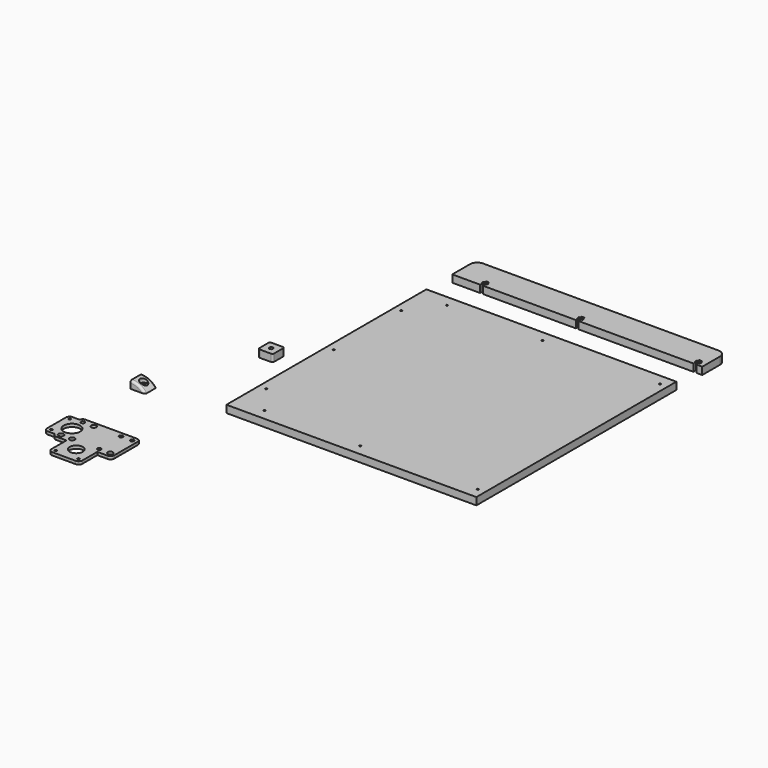
from build123d import *

# Parameters (mm, degrees)
F0_R          = 3.555
F0_R_2        = 1.5
F0_R_3        = 9
F0_R_4        = 11.2
F0_R_5        = 2.5
F1_DEPTH      = 4
F0_W          = 340
F0_H          = 340
F2_DEPTH      = 10
F6_DEPTH      = 39.1
F6_DEPTH_BACK = 25
F0_W_2        = 20
F0_H_2        = 20
F0_R_6        = 5
F8_DEPTH      = 10
F9_DEPTH      = 4
F11_DEPTH     = 25
F12_R         = 3
F13_D         = 2.5
F13_DEPTH     = 20
F13_TIP       = 0.7510757738
F14_DEPTH     = 10


# Not quite as in the source:
# - a feature of the source that left no trace in its solid (it failed there, or was rolled back) is left out
# - a feature names something its author has since deleted; it is built from what else it names


with BuildPart() as f1:
    # F0 (on Top) → F1 (new body)
    with BuildSketch(Plane.XY):
        with BuildLine():
            Line((35, 25), (-35, 25))
            ThreePointArc((-35, 25), (-38.1622776602, 23.8729833462), (-39.8989794856, 21))
            Line((-39.8989794856, 21), (-49.5, 21))
            ThreePointArc((-49.5, 21), (-53.0355339059, 19.5355339059), (-54.5, 16))
            Line((-54.5, 16), (-54.5, -16))
            ThreePointArc((-54.5, -16), (-53.0355339059, -19.5355339059), (-49.5, -21))
            Line((-49.5, -21), (-39.8989794856, -21))
            ThreePointArc((-39.8989794856, -21), (-38.1622776602, -23.8729833462), (-35, -25))
            Line((-35, -25), (-21, -25))
            Line((-21, -25), (-21, -50.5))
            ThreePointArc((-21, -50.5), (-19.5355339059, -54.0355339059), (-16, -55.5))
            Line((-16, -55.5), (16, -55.5))
            ThreePointArc((16, -55.5), (19.5355339059, -54.0355339059), (21, -50.5))
            Line((21, -50.5), (21, -25))
            Line((21, -25), (35, -25))
            ThreePointArc((35, -25), (38.5355339059, -23.5355339059), (40, -20))
            Line((40, -20), (40, 20))
            ThreePointArc((40, 20), (38.5355339059, 23.5355339059), (35, 25))
        make_face()
        with Locations((-33.5, -18.5)):
            Circle(F0_R, mode=Mode.SUBTRACT)
        with Locations((-15.5, -50)):
            Circle(F0_R_2, mode=Mode.SUBTRACT)
        with BuildLine():
            ThreePointArc((-21, -15.9725457472), (-17.1305977581, -15.2193350522), (-14.945, -18.5))
            ThreePointArc((-14.945, -18.5), (-17.1305977581, -21.7806649478), (-21, -21.0274542528))
            ThreePointArc((-21, -21.0274542528), (-22.055, -18.5), (-21, -15.9725457472))
        make_face(mode=Mode.SUBTRACT)
        with Locations((0, -34.5)):
            Circle(F0_R_3, mode=Mode.SUBTRACT)
        with Locations((-49, -15.5)):
            Circle(F0_R_2, mode=Mode.SUBTRACT)
        with Locations((-33.5, 0)):
            Circle(F0_R_4, mode=Mode.SUBTRACT)
        with Locations((-49, 15.5)):
            Circle(F0_R_2, mode=Mode.SUBTRACT)
        with Locations((-33.5, 18.5)):
            Circle(F0_R_5, mode=Mode.SUBTRACT)
        with Locations((-18.5, 18.5)):
            Circle(F0_R, mode=Mode.SUBTRACT)
        with Locations((15.5, -50)):
            Circle(F0_R_2, mode=Mode.SUBTRACT)
        with Locations((18.5, -18.5)):
            Circle(F0_R_5, mode=Mode.SUBTRACT)
        with Locations((33.5, -18.5)):
            Circle(F0_R, mode=Mode.SUBTRACT)
        with Locations((18.5, 18.5)):
            Circle(F0_R_5, mode=Mode.SUBTRACT)
        with Locations((33.5, 18.5)):
            Circle(F0_R_5, mode=Mode.SUBTRACT)
    extrude(amount=F1_DEPTH)

    # F5 (on Front) → F6 (cut, two sides)
    with BuildSketch(Plane.XZ) as f6_sk:
        with BuildLine():
            ThreePointArc((302.9023957253, 6.4145649905), (305.9114714076, 3.7905540573), (307.1651339531, 0))
            Line((307.1651339531, 0), (307.1651339531, 41.5010216767))
            Line((307.1651339531, 41.5010216767), (278.5302054882, 41.5010216767))
            ThreePointArc((278.5302054882, 41.5010216767), (286.2334403864, 20.8438533005), (302.9023957253, 6.4145649905))
        make_face()
    extrude(amount=F6_DEPTH, mode=Mode.SUBTRACT)
    extrude(f6_sk.sketch, amount=-F6_DEPTH_BACK, mode=Mode.SUBTRACT)


with BuildPart() as f2:
    # F0 (on Top) → F2 (new body)
    with BuildSketch(Plane.XY):
        with Locations((237.6083176136, 306.2372636795)):
            Rectangle(F0_W, F0_H)
    extrude(amount=F2_DEPTH)

    # F13
    with Locations(Plane(origin=(0, 0, 0), x_dir=(1, 0, 0), z_dir=(0, 0, -1))):
        with Locations((77.6083176136, -191.2372636795), (77.6083176136, -306.2372636795), (77.3551636471, -421.2380647742), (397.6083176136, -151.2372636795), (397.6083176136, -461.2372636795), (237.6083176136, -461.2372636795), (237.6083176136, -151.2372636795), (107.6083176136, -461.2372636795), (107.6083176136, -151.2372636795)):
            Hole(F13_D / 2, depth=F13_DEPTH)
            with Locations((0, 0, -(F13_DEPTH + F13_TIP / 2))):  # 118° drill point
                Cone(0, F13_D / 2, F13_TIP, mode=Mode.SUBTRACT)


with BuildPart() as f2b:
    # F0 (on Top) → F2, piece 2 (new body)
    with BuildSketch(Plane.XY):
        with BuildLine():
            Line((31, 277.586337328), (16, 277.586337328))
            ThreePointArc((16, 277.586337328), (14.232233047, 276.8541042809), (13.5, 275.086337328))
            Line((13.5, 275.086337328), (13.5, 260.086337328))
            ThreePointArc((13.5, 260.086337328), (14.232233047, 258.318570375), (16, 257.586337328))
            Line((16, 257.586337328), (31, 257.586337328))
            ThreePointArc((31, 257.586337328), (32.767766953, 258.318570375), (33.5, 260.086337328))
            Line((33.5, 260.086337328), (33.5, 275.086337328))
            ThreePointArc((33.5, 275.086337328), (32.767766953, 276.8541042809), (31, 277.586337328))
        make_face()
        with Locations((23.5, 267.586337328)):
            Circle(F0_R_5, mode=Mode.SUBTRACT)
    extrude(amount=F2_DEPTH)


with BuildPart() as f8:
    # F0 (on Top) → F8 (new body)
    with BuildSketch(Plane.XY):
        with Locations((-36.9331801683, 126.1065623164)):
            Rectangle(F0_W_2, F0_H_2)
        with Locations((-36.9331801683, 126.1065623164)):
            Circle(F0_R_6, mode=Mode.SUBTRACT)
    extrude(amount=F8_DEPTH)

    # F0 (on Top) → F9 (join)
    with BuildSketch(Plane.XY):
        with Locations((-36.9331801683, 126.1065623164)):
            Circle(F0_R_6)
        with Locations((-36.9331801683, 126.1065623164)):
            Circle(F0_R_5, mode=Mode.SUBTRACT)
    extrude(amount=F9_DEPTH)

    # F10 (on face) → F11 (cut)
    with BuildSketch(Plane.XZ.offset(-116.1065623164)):
        with BuildLine():
            ThreePointArc((-46.9331801683, 10), (-35.7528402808, 7.360679775), (-26.9331801683, 0))
            Line((-26.9331801683, 0), (-26.9331801683, 10))
            Line((-26.9331801683, 10), (-46.9331801683, 10))
        make_face()
    extrude(amount=-F11_DEPTH, mode=Mode.SUBTRACT)

    # F12
    f12_edges = [f8.edges().sort_by_distance(p)[0] for p in [
        (-35.75284, 116.106562, 7.36068),
        (-35.75284, 136.106562, 7.36068),
    ]]
    fillet(f12_edges, radius=F12_R)


with BuildPart() as f14:
    # F0 (on Top) → F14 (new body)
    with BuildSketch(Plane.XY):
        with BuildLine():
            Line((67.6083176136, 550.2482438087), (67.6083176136, 520.2482438087))
            Line((67.6083176136, 520.2482438087), (105.6083176136, 520.2482438087))
            Line((105.6083176136, 520.2482438087), (105.6083176136, 524.423217392))
            Line((105.6083176136, 524.423217392), (104.1083176136, 524.423217392))
            Line((104.1083176136, 524.423217392), (104.1083176136, 527.723217392))
            Line((104.1083176136, 527.723217392), (105.6083176136, 527.723217392))
            Line((105.6083176136, 527.723217392), (105.6083176136, 530.2482438087))
            Line((105.6083176136, 530.2482438087), (109.6083176136, 530.2482438087))
            Line((109.6083176136, 530.2482438087), (109.6083176136, 527.723217392))
            Line((109.6083176136, 527.723217392), (111.1083176136, 527.723217392))
            Line((111.1083176136, 527.723217392), (111.1083176136, 524.423217392))
            Line((111.1083176136, 524.423217392), (109.6083176136, 524.423217392))
            Line((109.6083176136, 524.423217392), (109.6083176136, 520.2482438087))
            Line((109.6083176136, 520.2482438087), (235.6083176136, 520.2482438087))
            Line((235.6083176136, 520.2482438087), (235.6083176136, 524.423217392))
            Line((235.6083176136, 524.423217392), (234.1083176136, 524.423217392))
            Line((234.1083176136, 524.423217392), (234.1083176136, 527.723217392))
            Line((234.1083176136, 527.723217392), (235.6083176136, 527.723217392))
            Line((235.6083176136, 527.723217392), (235.6083176136, 530.2482438087))
            Line((235.6083176136, 530.2482438087), (239.6083176136, 530.2482438087))
            Line((239.6083176136, 530.2482438087), (239.6083176136, 527.723217392))
            Line((239.6083176136, 527.723217392), (241.1083176136, 527.723217392))
            Line((241.1083176136, 527.723217392), (241.1083176136, 524.423217392))
            Line((241.1083176136, 524.423217392), (239.6083176136, 524.423217392))
            Line((239.6083176136, 524.423217392), (239.6083176136, 520.2482438087))
            Line((239.6083176136, 520.2482438087), (395.6083176136, 520.2482438087))
            Line((395.6083176136, 520.2482438087), (395.6083176136, 524.423217392))
            Line((395.6083176136, 524.423217392), (394.1083176136, 524.423217392))
            Line((394.1083176136, 524.423217392), (394.1083176136, 527.723217392))
            Line((394.1083176136, 527.723217392), (395.6083176136, 527.723217392))
            Line((395.6083176136, 527.723217392), (395.6083176136, 530.2482438087))
            Line((395.6083176136, 530.2482438087), (399.6083176136, 530.2482438087))
            Line((399.6083176136, 530.2482438087), (399.6083176136, 527.723217392))
            Line((399.6083176136, 527.723217392), (401.1083176136, 527.723217392))
            Line((401.1083176136, 527.723217392), (401.1083176136, 524.423217392))
            Line((401.1083176136, 524.423217392), (399.6083176136, 524.423217392))
            Line((399.6083176136, 524.423217392), (399.6083176136, 520.2482438087))
            Line((399.6083176136, 520.2482438087), (407.6083176136, 520.2482438087))
            Line((407.6083176136, 520.2482438087), (407.6083176136, 550.2482438087))
            ThreePointArc((407.6083176136, 550.2482438087), (404.6793854255, 557.3193116206), (397.6083176136, 560.2482438087))
            Line((397.6083176136, 560.2482438087), (77.6083176136, 560.2482438087))
            ThreePointArc((77.6083176136, 560.2482438087), (70.5372498017, 557.3193116206), (67.6083176136, 550.2482438087))
        make_face()
    extrude(amount=F14_DEPTH)


solid = Compound([f1.part, f2.part, f2b.part, f8.part, f14.part])
